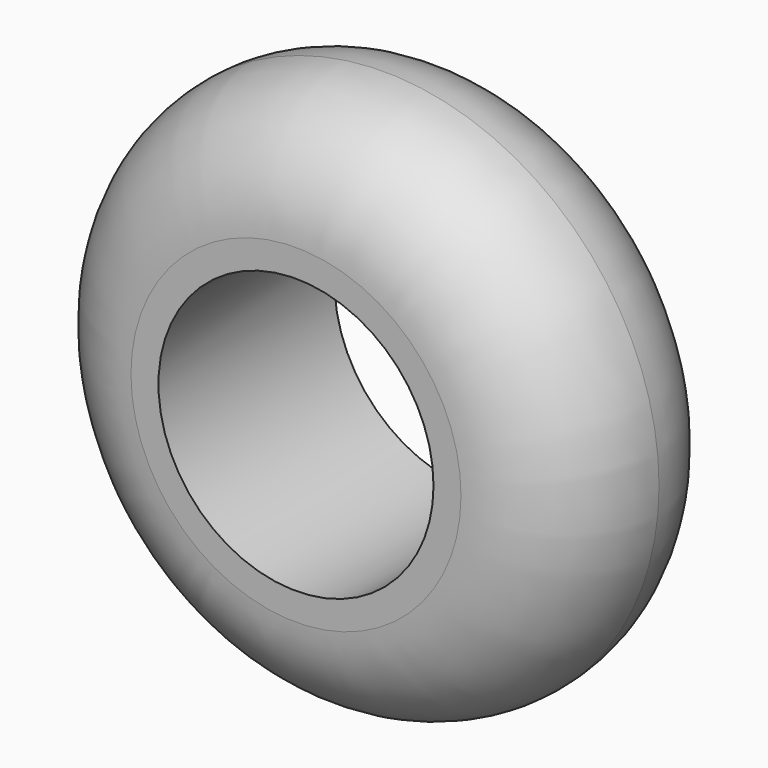
from build123d import *

# Parameters (mm, degrees)
F0_R     = 15.875
F0_R_2   = 7.9375
F1_DEPTH = 12.7
F2_R     = 6.34999


# Not quite as in the source:
# - a fillet or chamfer is up to 0.001 mm smaller than in the source, because OpenCascade refuses the exact size


with BuildPart() as f1:
    # F0 (on Front) → F1 (new body)
    with BuildSketch(Plane.XZ):
        with Locations((-29.4404756278, 24.1331793368)):
            Circle(F0_R)
        with Locations((-29.4404756278, 24.1331793368)):
            Circle(F0_R_2, mode=Mode.SUBTRACT)
    extrude(amount=F1_DEPTH)

    # F2 (radius 6.35 in the source; OpenCascade refuses exactly that, so slightly less here)
    f2_edges = [f1.edges().sort_by_distance(p)[0] for p in [
        (-45.315476, -12.7, 24.133179),
        (-45.315476, 0, 24.133179),
    ]]
    fillet(f2_edges, radius=F2_R)


solid = f1.part
